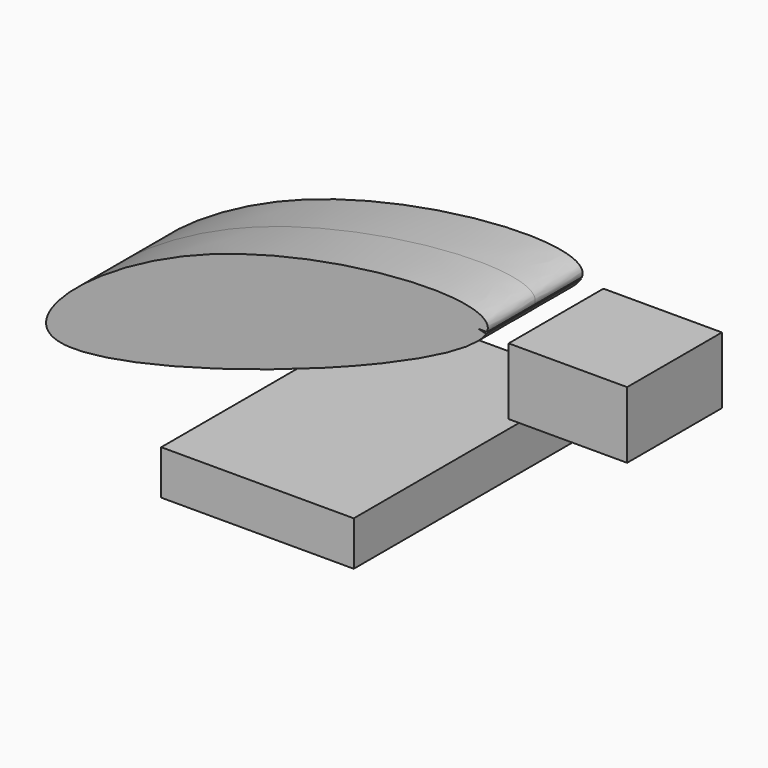
from build123d import *

# Parameters (mm, degrees)
F1_DEPTH = 63.5
F2_DEPTH = 25.4
F3_DEPTH = 25.4


with BuildPart() as f1:
    # F0 (on Front) → F1 (new body, symmetric)
    with BuildSketch(Plane.XZ):
        Polygon((-41.275, -9.525), (41.275, -9.525), (41.275, 9.525), (22.225, 9.525), (-41.275, 9.525), align=None)
    extrude(amount=F1_DEPTH, both=True)


with BuildPart() as f2:
    # F0 (on Front) → F2 (new body, symmetric)
    with BuildSketch(Plane.XZ):
        with BuildLine():
            add(Edge.make_bspline(
                [(-116.5613234043, 9.9720694125), (-98.6556275911, 4.555359494), (-25.5967653083, 26.1168675806), (23.1180103528, 46.6597712092)],
                knots=[0, 0, 0, 0, 0.278306286, 0.278306286, 0.278306286, 0.278306286], degree=3))
            ThreePointArc((23.1180103528, 46.6597712092), (38.2764501263, 68.1986546895), (64.1686919931, 73.025))
            Line((64.1686919931, 73.025), (67.9254966229, 73.025))
            add(Edge.make_bspline(
                [(67.9254966229, 73.025), (73.9295375569, 87.6886672071), (-61.9721796473, 79.771290711), (-133.432077068, 15.075695636), (-116.5613234043, 9.9720694125)],
                knots=[0.4160907456, 0.4160907456, 0.4160907456, 0.4160907456, 0.7377797075, 1, 1, 1, 1], degree=3))
        make_face()
    extrude(amount=F2_DEPTH, both=True)

    # F0 (on Front) → F3, piece 2 (join, symmetric)
    with BuildSketch(Plane.XZ):
        with BuildLine():
            ThreePointArc((64.1686919931, 73.025), (38.2764501263, 68.1986546895), (23.1180103528, 46.6597712092))
            add(Edge.make_bspline(
                [(23.1180103528, 46.6597712092), (46.1676927195, 56.3797667772), (63.7673065848, 65.8717207614), (67.4958292711, 72.1699724917)],
                knots=[0.278306286, 0.278306286, 0.278306286, 0.278306286, 0.4099885406, 0.4099885406, 0.4099885406, 0.4099885406], degree=3))
            ThreePointArc((67.4958292711, 72.1699724917), (65.8427796299, 72.6384184373), (64.1686919931, 73.025))
        make_face()
    extrude(amount=F3_DEPTH, both=True)


with BuildPart() as f3:
    # F0 (on Front) → F3 (new body, symmetric)
    with BuildSketch(Plane.XZ):
        Polygon((77.1917359352, 71.755), (77.1917359352, 53.975), (77.1917359352, 43.18), (127.9917359352, 43.18), (127.9917359352, 71.755), align=None)
    extrude(amount=F3_DEPTH, both=True)


solid = Compound([f1.part, f2.part, f3.part])
